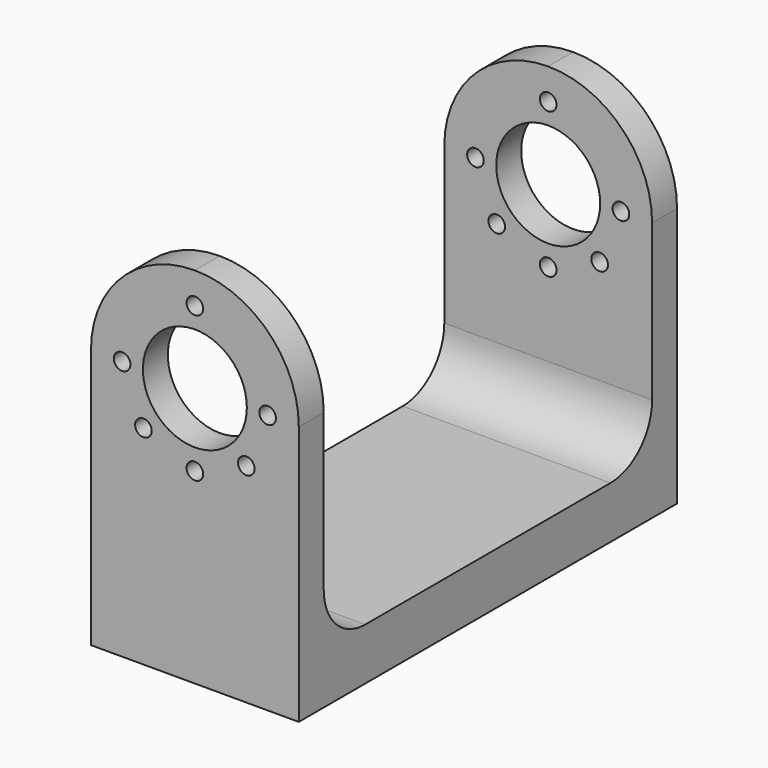
from build123d import *

# Parameters (mm, degrees)
F0_R     = 0.8
F0_R_2   = 5
F1_DEPTH = 45.5
F2_W     = 39.5
F2_H     = 30
F3_DEPTH = 20.001
F4_DEPTH = 45.501
F5_R     = 5


with BuildPart() as f1:
    # F0 (on Front) → F1 (new body)
    with BuildSketch(Plane.XZ):
        with BuildLine():
            ThreePointArc((-2.67e-08, 10), (-7.0710678213, 7.0710678024), (-10, 0))
            ThreePointArc((-10, 0), (0, -10), (10, 0))
            ThreePointArc((10, 0), (7.0710678024, 7.0710678213), (-2.67e-08, 10))
        make_face()
        with Locations((-7, 0)):
            Circle(F0_R, mode=Mode.SUBTRACT)
        with Locations((-4.9497474683, -4.9497474683)):
            Circle(F0_R, mode=Mode.SUBTRACT)
        with Locations((0, -7)):
            Circle(F0_R, mode=Mode.SUBTRACT)
        with Locations((4.9497474683, -4.9497474683)):
            Circle(F0_R, mode=Mode.SUBTRACT)
        Circle(F0_R_2, mode=Mode.SUBTRACT)
        with Locations((7, 0)):
            Circle(F0_R, mode=Mode.SUBTRACT)
        with Locations((0, 7)):
            Circle(F0_R, mode=Mode.SUBTRACT)
        with BuildLine():
            ThreePointArc((10, 0), (0, -10), (-10, 0))
            Line((-10, 0), (-10, -22))
            Line((-10, -22), (10, -22))
            Line((10, -22), (10, 0))
        make_face()
        Circle(F0_R_2)
        Polygon((10, -22), (-10, -22), (-10, -25), (0, -25), (10, -25), align=None)
        with BuildLine():
            ThreePointArc((-2.67e-08, 10), (7.0710678024, 7.0710678213), (10, 0))
            Line((10, 0), (10, 10))
            Line((10, 10), (-2.67e-08, 10))
        make_face()
        with BuildLine():
            Line((-10, 10), (-10, 0))
            ThreePointArc((-10, 0), (-7.0710678213, 7.0710678024), (-2.67e-08, 10))
            Line((-2.67e-08, 10), (-10, 10))
        make_face()
        with Locations((0, -7)):
            Circle(F0_R)
        with Locations((7, 0)):
            Circle(F0_R)
        with Locations((-4.9497474683, -4.9497474683)):
            Circle(F0_R)
        with Locations((-7, 0)):
            Circle(F0_R)
        with Locations((0, 7)):
            Circle(F0_R)
        with Locations((4.9497474683, -4.9497474683)):
            Circle(F0_R)
    extrude(amount=-F1_DEPTH)

    # F2 (on face) → F3 (cut, through all)
    with BuildSketch(Plane.YZ.offset(10)):
        with Locations((22.75, -5)):
            Rectangle(F2_W, F2_H)
    extrude(amount=-F3_DEPTH, mode=Mode.SUBTRACT)

    # F0 (on Front) → F4 (cut, through all)
    with BuildSketch(Plane.XZ):
        Circle(F0_R_2)
        with BuildLine():
            Line((-10, 10), (-10, 0))
            ThreePointArc((-10, 0), (-7.0710678213, 7.0710678024), (-2.67e-08, 10))
            Line((-2.67e-08, 10), (-10, 10))
        make_face()
        with BuildLine():
            ThreePointArc((-2.67e-08, 10), (7.0710678024, 7.0710678213), (10, 0))
            Line((10, 0), (10, 10))
            Line((10, 10), (-2.67e-08, 10))
        make_face()
        with Locations((7, 0)):
            Circle(F0_R)
        with Locations((0, 7)):
            Circle(F0_R)
        with Locations((-7, 0)):
            Circle(F0_R)
        with Locations((-4.9497474683, -4.9497474683)):
            Circle(F0_R)
        with Locations((0, -7)):
            Circle(F0_R)
        with Locations((4.9497474683, -4.9497474683)):
            Circle(F0_R)
    extrude(amount=-F4_DEPTH, mode=Mode.SUBTRACT)

    # F5
    f5_edges = [f1.edges().sort_by_distance(p)[0] for p in [
        (0, 42.5, -20),
        (0, 3, -20),
    ]]
    fillet(f5_edges, radius=F5_R)


solid = f1.part
